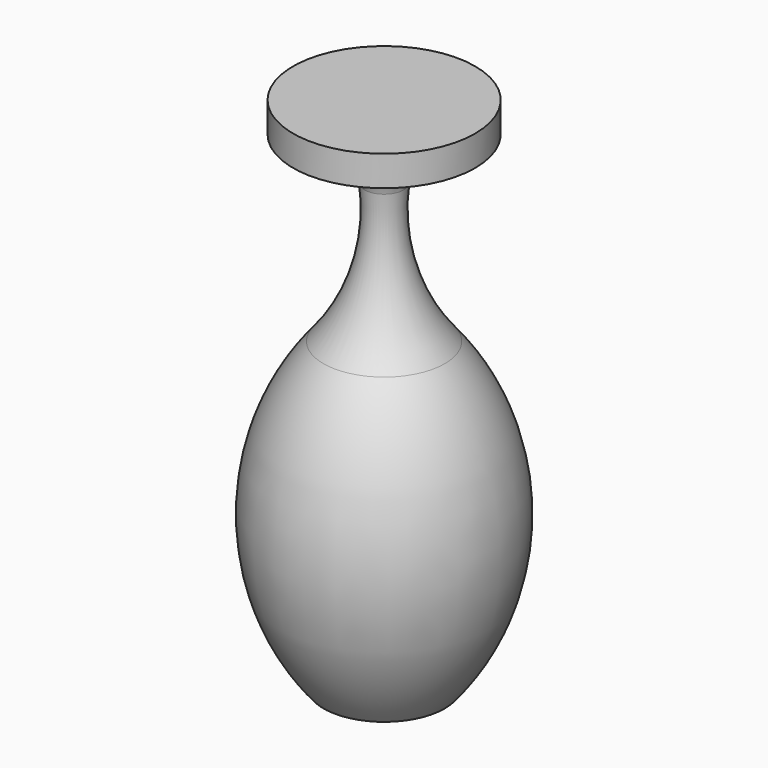
from build123d import *

# Parameters (mm, degrees)
F2_R = 8


with BuildPart() as f1:
    # F0 (on Front) → F1 (revolve)
    with BuildSketch(Plane.XZ):
        with BuildLine():
            Line((0, 80), (0, 0))
            Line((0, 0), (10, 0))
            ThreePointArc((10, 0), (19.079415133, 25), (10, 50))
            ThreePointArc((10, 50), (3.4165275014, 64.3194212502), (5, 80))
            Line((5, 80), (15, 80))
            Line((15, 80), (15, 85))
            Line((15, 85), (0, 85))
            Line((0, 85), (0, 80))
        make_face()
    revolve(axis=Axis((0, 0, 40), (0, 0, 1)))

    # F2
    f2_edges = [f1.edges().sort_by_distance(p)[0] for p in [
        (-5, 0, 80),
    ]]
    fillet(f2_edges, radius=F2_R)


solid = f1.part
